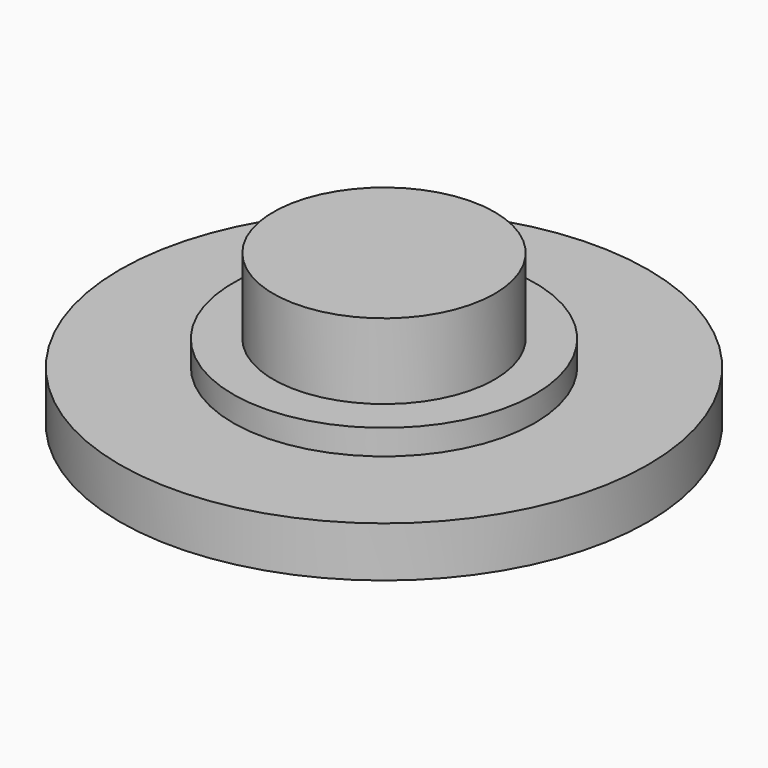
from build123d import *

# Parameters (mm, degrees)
F0_R         = 10.5
F1_DEPTH     = 2
F2_R         = 6
F3_DEPTH     = 1
F4_R         = 4.4
F5_DEPTH     = 3
F6_TEXT_SIZE = 22.7162069177
F7_DEPTH     = 1


# Not quite as in the source:
# - Text() gives the source's letters only with a copy of the font that has no kerning and outlines rounded to 1/6400 em; it was checked with that copy


with BuildPart() as f1:
    # F0 (on Top) → F1 (new body)
    with BuildSketch(Plane.XY):
        Circle(F0_R)
    extrude(amount=F1_DEPTH)

    # F2 (on face) → F3 (join)
    with BuildSketch(Plane.XY.offset(2)):
        Circle(F2_R)
    extrude(amount=F3_DEPTH)

    # F4 (on face) → F5 (join)
    with BuildSketch(Plane.XY.offset(3)):
        Circle(F4_R)
    extrude(amount=F5_DEPTH)

    # F6 (on face) → F7 (cut)
    with BuildSketch(Plane(origin=(0, 0, 0), x_dir=(1, 0, 0), z_dir=(0, 0, -1))):
        with Locations((-6.5008449827, -8.1778344904)):
            Text('S', F6_TEXT_SIZE, font='Open Sans', font_style=FontStyle.BOLD, text_align=(TextAlign.LEFT, TextAlign.BOTTOM))
    extrude(amount=-F7_DEPTH, mode=Mode.SUBTRACT)


solid = f1.part
